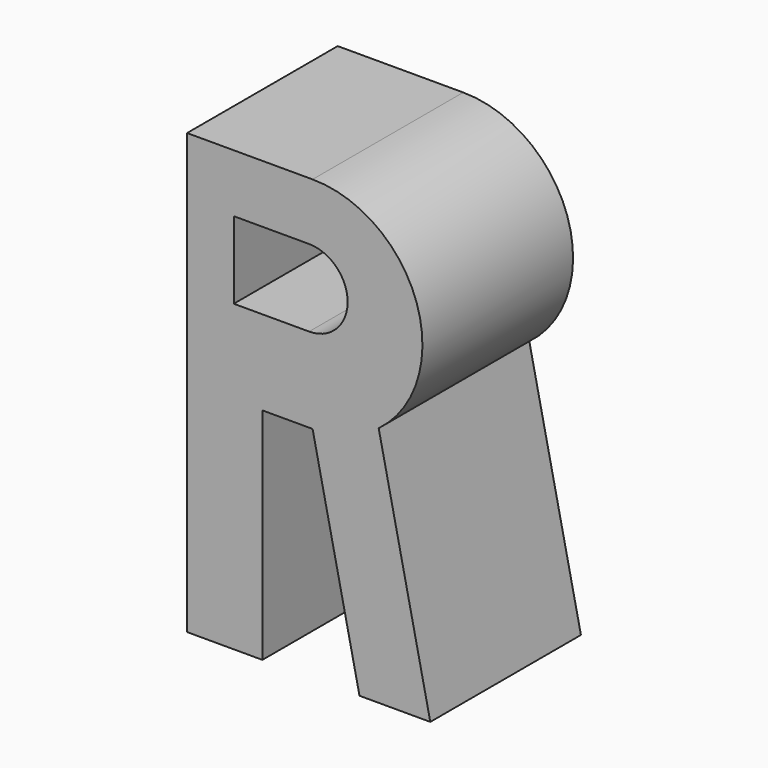
from build123d import *

# Parameters (mm, degrees)
F0_W     = 3.048
F0_H     = 8.89
F1_DEPTH = 7.62
F2_DEPTH = 7.62
F3_W     = 3.048
F3_H     = 3.1197171271
F4_DEPTH = 25.4


# Not quite as in the source:
# - a feature names something its author has since deleted; it is built from what else it names


with BuildPart() as f1:
    # F0 (on Front) → F1 (new body)
    with BuildSketch(Plane.XZ):
        Polygon((-6.9585410112, 8.89), (-12.0385410112, 8.89), (-12.0385410112, 0), (-8.9905410112, 0), (-6.9585410112, 0), align=None)
        with BuildLine():
            ThreePointArc((-4.2838060673, 0.8948143739), (-2.7431762518, 5.8552215946), (-6.9585410112, 8.89))
            Line((-6.9585410112, 8.89), (-6.9585410112, 0))
            ThreePointArc((-6.9585410112, 0), (-5.5483194165, 0.2296352407), (-4.2838060673, 0.8948143739))
        make_face()
        with Locations((-10.5145410112, -4.445)):
            Rectangle(F0_W, F0_H)
    extrude(amount=F1_DEPTH)

    # F0 (on Front) → F2 (join)
    with BuildSketch(Plane.XZ):
        Polygon((-6.9585410112, 8.89), (-12.0385410112, 8.89), (-12.0385410112, 0), (-8.9905410112, 0), (-6.9585410112, 0), align=None)
        with BuildLine():
            ThreePointArc((-4.2838060673, 0.8948143739), (-2.7431762518, 5.8552215946), (-6.9585410112, 8.89))
            Line((-6.9585410112, 8.89), (-6.9585410112, 0))
            ThreePointArc((-6.9585410112, 0), (-5.5483194165, 0.2296352407), (-4.2838060673, 0.8948143739))
        make_face()
        with Locations((-10.5145410112, -4.445)):
            Rectangle(F0_W, F0_H)
        with BuildLine():
            ThreePointArc((-4.2838060673, 0.8948143739), (-5.5483194165, 0.2296352407), (-6.9585410112, 0))
            Line((-6.9585410112, 0), (-5.0608660094, -8.89))
            Line((-5.0608660094, -8.89), (-2.1951224189, -8.89))
            Line((-2.1951224189, -8.89), (-4.2838060673, 0.8948143739))
        make_face()
    extrude(amount=F2_DEPTH)

    # F3 (on face) → F4 (cut)
    with BuildSketch(Plane.XZ.offset(7.62)):
        with Locations((-8.624184413, 4.9824524904)):
            Rectangle(F3_W, F3_H)
        with BuildLine():
            ThreePointArc((-7.100184413, 3.4225939268), (-5.5403258494, 4.9824524904), (-7.100184413, 6.5423110539))
            Line((-7.100184413, 6.5423110539), (-7.100184413, 3.4225939268))
        make_face()
    extrude(amount=-F4_DEPTH, mode=Mode.SUBTRACT)


solid = f1.part
